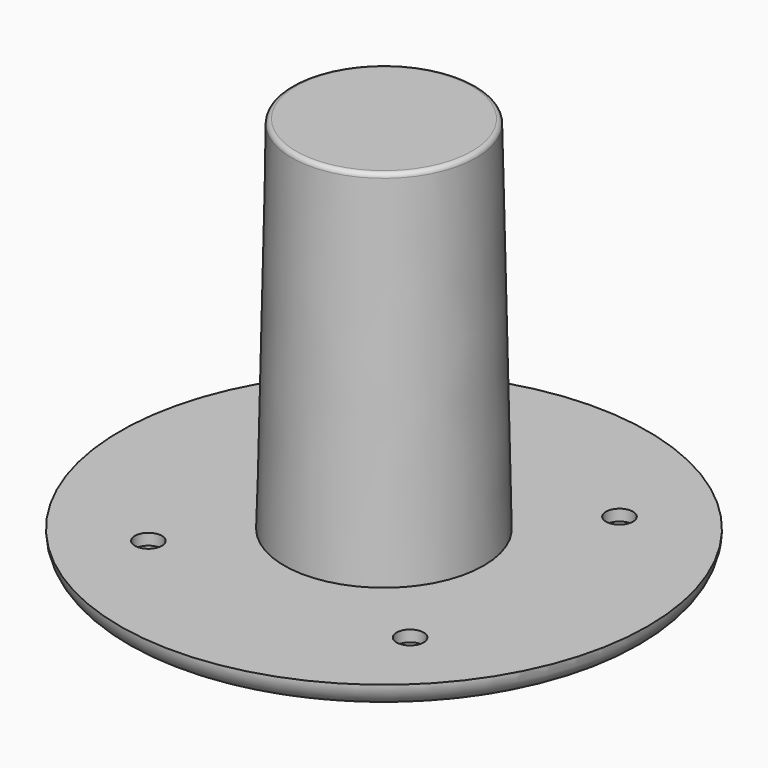
from build123d import *

# Parameters (mm, degrees)
F0_R           = 22.25
F0_R_2         = 21.25
F1_DEPTH       = 85.5
F1_TAPER       = 1.2
F2_T           = -4
F0_R_3         = 58.5
F0_R_4         = 3
F3_DEPTH       = 5.5
F4_R           = 5.49999
F5_D           = 6
F5_DEPTH       = 5
F5_CBORE_D     = 10
F5_CBORE_DEPTH = 3
F5_TIP         = 1.8025818571
F6_R           = 1
F7_R           = 3


# Not quite as in the source:
# - a fillet or chamfer is up to 0.001 mm smaller than in the source, because OpenCascade refuses the exact size


with BuildPart() as f1:
    # F0 (on Top) → F1 (new body)
    with BuildSketch(Plane.XY):
        Circle(F0_R)
        Circle(F0_R_2, mode=Mode.SUBTRACT)
        Circle(F0_R_2)
    extrude(amount=F1_DEPTH, taper=F1_TAPER)

    # F2
    f2_openings = [f1.faces().sort_by_distance(p)[0] for p in [
        (0, 0, 0),
    ]]
    offset(amount=F2_T, openings=f2_openings)

    # F0 (on Top) → F3 (join)
    with BuildSketch(Plane.XY):
        Circle(F0_R_3)
        with Locations((-29, -29)):
            Circle(F0_R_4, mode=Mode.SUBTRACT)
        with Locations((29, -29)):
            Circle(F0_R_4, mode=Mode.SUBTRACT)
        with Locations((-29, 29)):
            Circle(F0_R_4, mode=Mode.SUBTRACT)
        Circle(F0_R, mode=Mode.SUBTRACT)
        with Locations((29, 29)):
            Circle(F0_R_4, mode=Mode.SUBTRACT)
        Circle(F0_R)
        Circle(F0_R_2, mode=Mode.SUBTRACT)
    extrude(amount=F3_DEPTH)

    # F4 (radius 5.5 in the source; OpenCascade refuses exactly that, so slightly less here)
    f4_edges = [f1.edges().sort_by_distance(p)[0] for p in [
        (-58.5, 0, 0),
    ]]
    fillet(f4_edges, radius=F4_R)

    # F5
    with Locations(Plane(origin=(0, 0, 0), x_dir=(1, 0, 0), z_dir=(0, 0, -1))):
        with Locations((29, -29), (-29, -29), (-29, 29), (29, 29)):
            CounterBoreHole(F5_D / 2, F5_CBORE_D / 2, F5_CBORE_DEPTH, depth=F5_DEPTH)
            with Locations((0, 0, -(F5_DEPTH + F5_TIP / 2))):  # 118° drill point
                Cone(0, F5_D / 2, F5_TIP, mode=Mode.SUBTRACT)

    # F6
    f6_edges = [f1.edges().sort_by_distance(p)[0] for p in [
        (-20.45903, 0, 85.5),
    ]]
    fillet(f6_edges, radius=F6_R)

    # F7
    f7_edges = [f1.edges().sort_by_distance(p)[0] for p in [
        (-18.249123, 0, 0),
    ]]
    fillet(f7_edges, radius=F7_R)


solid = f1.part
